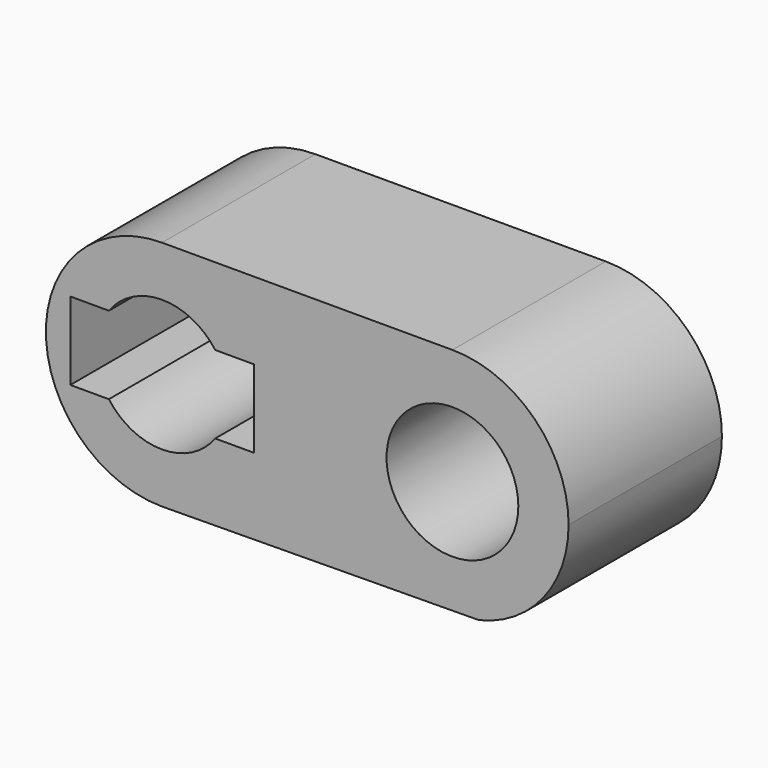
from build123d import *

# Parameters (mm, degrees)
F0_R     = 14.4101824993
F1_DEPTH = 41.91
F4_DEPTH = 119.38


# Not quite as in the source:
# - a feature of the source that left no trace in its solid (it failed there, or was rolled back) is left out


with BuildPart() as f1:
    # F0 (on Front) → F1 (new body)
    with BuildSketch(Plane.XZ):
        with BuildLine():
            ThreePointArc((0.4902951327, -25.3952674859), (18.133029206, -17.7863220429), (25.4, 0))
            ThreePointArc((25.4, 0), (17.9605122421, 17.9605122421), (0, 25.4))
            ThreePointArc((0, 25.4), (-25.4, 0), (0, -25.4))
            Line((0, -25.4), (0.4902951327, -25.3952674859))
        make_face()
        with BuildLine():
            ThreePointArc((-11.6233856549, 8.5176443681), (0, 14.4101824993), (11.6233856549, 8.5176443681))
            Line((11.6233856549, 8.5176443681), (20.0593080372, 8.5176443681))
            Line((20.0593080372, 8.5176443681), (20.0593080372, -8.5176443681))
            Line((20.0593080372, -8.5176443681), (11.6233856549, -8.5176443681))
            ThreePointArc((11.6233856549, -8.5176443681), (0, -14.4101824993), (-11.6233856549, -8.5176443681))
            Line((-11.6233856549, -8.5176443681), (-20.0593080372, -8.5176443681))
            Line((-20.0593080372, -8.5176443681), (-20.0593080372, 8.5176443681))
            Line((-20.0593080372, 8.5176443681), (-11.6233856549, 8.5176443681))
        make_face(mode=Mode.SUBTRACT)
        with BuildLine():
            ThreePointArc((0, 25.4), (17.9605122421, 17.9605122421), (25.4, 0))
            ThreePointArc((25.4, 0), (18.133029206, -17.7863220429), (0.4902951327, -25.3952674859))
            Line((0.4902951327, -25.3952674859), (58.1880762297, -24.8383466813))
            ThreePointArc((58.1880762297, -24.8383466813), (38.2408035984, 2.670767146), (63.5, 25.4))
            Line((63.5, 25.4), (0, 25.4))
        make_face()
        with BuildLine():
            ThreePointArc((88.9, 0), (81.4605122421, 17.9605122421), (63.5, 25.4))
            ThreePointArc((63.5, 25.4), (38.2408035984, 2.670767146), (58.1880762297, -24.8383466813))
            Line((58.1880762297, -24.8383466813), (69.2903876179, -24.7311829728))
            ThreePointArc((69.2903876179, -24.7311829728), (83.4027114421, -15.7810670505), (88.9, 0))
        make_face()
        with Locations((63.5, 0)):
            Circle(F0_R, mode=Mode.SUBTRACT)
        with Locations((63.5, 0)):
            Circle(F0_R)
        with BuildLine():
            ThreePointArc((-11.6233856549, -8.5176443681), (-14.4101824993, 0), (-11.6233856549, 8.5176443681))
            Line((-11.6233856549, 8.5176443681), (-20.0593080372, 8.5176443681))
            Line((-20.0593080372, 8.5176443681), (-20.0593080372, -8.5176443681))
            Line((-20.0593080372, -8.5176443681), (-11.6233856549, -8.5176443681))
        make_face()
        with BuildLine():
            ThreePointArc((11.6233856549, -8.5176443681), (13.6957743156, -4.4809737288), (14.4101824993, 0))
            ThreePointArc((14.4101824993, 0), (13.6957743156, 4.4809737288), (11.6233856549, 8.5176443681))
            Line((11.6233856549, 8.5176443681), (-11.6233856549, 8.5176443681))
            ThreePointArc((-11.6233856549, 8.5176443681), (-14.4101824993, 0), (-11.6233856549, -8.5176443681))
            Line((-11.6233856549, -8.5176443681), (11.6233856549, -8.5176443681))
        make_face()
        with BuildLine():
            Line((-11.6233856549, 8.5176443681), (11.6233856549, 8.5176443681))
            ThreePointArc((11.6233856549, 8.5176443681), (0, 14.4101824993), (-11.6233856549, 8.5176443681))
        make_face()
        with BuildLine():
            ThreePointArc((-11.6233856549, -8.5176443681), (0, -14.4101824993), (11.6233856549, -8.5176443681))
            Line((11.6233856549, -8.5176443681), (-11.6233856549, -8.5176443681))
        make_face()
        with BuildLine():
            ThreePointArc((11.6233856549, 8.5176443681), (13.6957743156, 4.4809737288), (14.4101824993, 0))
            ThreePointArc((14.4101824993, 0), (13.6957743156, -4.4809737288), (11.6233856549, -8.5176443681))
            Line((11.6233856549, -8.5176443681), (20.0593080372, -8.5176443681))
            Line((20.0593080372, -8.5176443681), (20.0593080372, 8.5176443681))
            Line((20.0593080372, 8.5176443681), (11.6233856549, 8.5176443681))
        make_face()
    extrude(amount=-F1_DEPTH)

    # F0 (on Front) → F4 (cut)
    with BuildSketch(Plane.XZ):
        with BuildLine():
            ThreePointArc((-11.6233856549, -8.5176443681), (-14.4101824993, 0), (-11.6233856549, 8.5176443681))
            Line((-11.6233856549, 8.5176443681), (-20.0593080372, 8.5176443681))
            Line((-20.0593080372, 8.5176443681), (-20.0593080372, -8.5176443681))
            Line((-20.0593080372, -8.5176443681), (-11.6233856549, -8.5176443681))
        make_face()
        with BuildLine():
            Line((-11.6233856549, 8.5176443681), (11.6233856549, 8.5176443681))
            ThreePointArc((11.6233856549, 8.5176443681), (0, 14.4101824993), (-11.6233856549, 8.5176443681))
        make_face()
        with BuildLine():
            ThreePointArc((11.6233856549, 8.5176443681), (13.6957743156, 4.4809737288), (14.4101824993, 0))
            ThreePointArc((14.4101824993, 0), (13.6957743156, -4.4809737288), (11.6233856549, -8.5176443681))
            Line((11.6233856549, -8.5176443681), (20.0593080372, -8.5176443681))
            Line((20.0593080372, -8.5176443681), (20.0593080372, 8.5176443681))
            Line((20.0593080372, 8.5176443681), (11.6233856549, 8.5176443681))
        make_face()
        with BuildLine():
            ThreePointArc((11.6233856549, -8.5176443681), (13.6957743156, -4.4809737288), (14.4101824993, 0))
            ThreePointArc((14.4101824993, 0), (13.6957743156, 4.4809737288), (11.6233856549, 8.5176443681))
            Line((11.6233856549, 8.5176443681), (-11.6233856549, 8.5176443681))
            ThreePointArc((-11.6233856549, 8.5176443681), (-14.4101824993, 0), (-11.6233856549, -8.5176443681))
            Line((-11.6233856549, -8.5176443681), (11.6233856549, -8.5176443681))
        make_face()
        with BuildLine():
            ThreePointArc((-11.6233856549, -8.5176443681), (0, -14.4101824993), (11.6233856549, -8.5176443681))
            Line((11.6233856549, -8.5176443681), (-11.6233856549, -8.5176443681))
        make_face()
        with Locations((63.5, 0)):
            Circle(F0_R)
    extrude(amount=-F4_DEPTH, mode=Mode.SUBTRACT)


solid = f1.part
